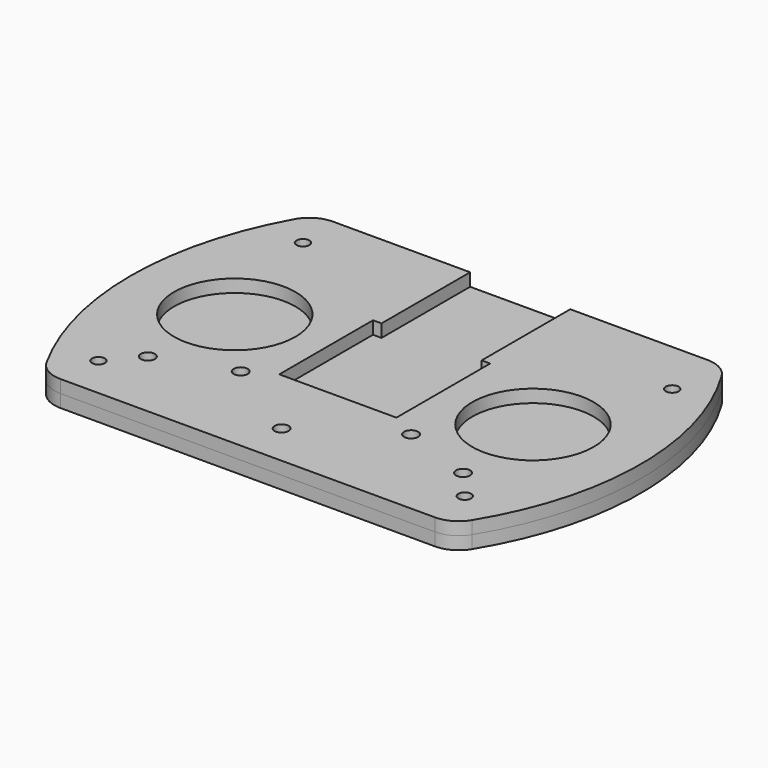
from build123d import *

# Parameters (mm, degrees)
F0_R     = 1.5
F1_DEPTH = 3
F2_DEPTH = 3
F3_R     = 14.25
F3_R_2   = 1.65
F4_DEPTH = 25
F6_DEPTH = 3
F7_DEPTH = 3
F8_W     = 23.5
F8_H     = 37.6963340342
F9_DEPTH = 25


with BuildPart() as f1:
    # F0 (on Top) → F1 (new body)
    with BuildSketch(Plane.XY):
        with BuildLine():
            Line((45.1, 35), (-45.1, 35))
            ThreePointArc((-45.1, 35), (-54.4782217351, 0), (-45.1, -35))
            Line((-45.1, -35), (45.1, -35))
            ThreePointArc((45.1, -35), (55.2720579016, 0), (45.1, 35))
        make_face()
        with Locations((-43, -30)):
            Circle(F0_R, mode=Mode.SUBTRACT)
        with Locations((43, -30)):
            Circle(F0_R, mode=Mode.SUBTRACT)
        with Locations((-43, 30)):
            Circle(F0_R, mode=Mode.SUBTRACT)
        with Locations((46.13, 26.95)):
            Circle(F0_R, mode=Mode.SUBTRACT)
    extrude(amount=-F1_DEPTH)

    # F5 (on Top) → F6 (join)
    with BuildSketch(Plane.XY):
        with BuildLine():
            ThreePointArc((-50.0545445124, 36.3970588235), (-59.4782217351, 0), (-50.0545445124, -36.3970588235))
            ThreePointArc((-50.0545445124, -36.3970588235), (-47.4851853132, -39.0323880746), (-43.9340877199, -40))
            Line((-43.9340877199, -40), (43.9895550669, -40))
            ThreePointArc((43.9895550669, -40), (47.4140971022, -39.1051217718), (49.9630539635, -36.6492890995))
            ThreePointArc((49.9630539635, -36.6492890995), (60.2720579016, 0), (49.9630539635, 36.6492890995))
            ThreePointArc((49.9630539635, 36.6492890995), (47.4140971022, 39.1051217718), (43.9895550669, 40))
            Line((43.9895550669, 40), (-43.9340877199, 40))
            ThreePointArc((-43.9340877199, 40), (-47.4851853132, 39.0323880746), (-50.0545445124, 36.3970588235))
        make_face()
        with BuildLine():
            Line((44.5476018751, -34), (-44.5198739442, -34))
            ThreePointArc((-44.5198739442, -34), (-53.4782217351, 0), (-44.5198739442, 34))
            Line((-44.5198739442, 34), (44.5476018751, 34))
            ThreePointArc((44.5476018751, 34), (54.2720579016, 0), (44.5476018751, -34))
        make_face(mode=Mode.SUBTRACT)
    extrude(amount=-F6_DEPTH)


with BuildPart() as f2:
    # F0 (on Top) → F2 (new body)
    with BuildSketch(Plane.XY):
        with BuildLine():
            Line((45.1, 35), (-45.1, 35))
            ThreePointArc((-45.1, 35), (-54.4782217351, 0), (-45.1, -35))
            Line((-45.1, -35), (45.1, -35))
            ThreePointArc((45.1, -35), (55.2720579016, 0), (45.1, 35))
        make_face()
        with Locations((-43, -30)):
            Circle(F0_R, mode=Mode.SUBTRACT)
        with Locations((43, -30)):
            Circle(F0_R, mode=Mode.SUBTRACT)
        with Locations((-43, 30)):
            Circle(F0_R, mode=Mode.SUBTRACT)
        with Locations((46.13, 26.95)):
            Circle(F0_R, mode=Mode.SUBTRACT)
    extrude(amount=F2_DEPTH)

    # F3 (on Top) → F4 (cut)
    with BuildSketch(Plane.XY):
        Polygon((-11.75, 14), (-13.75, 14), (-13.75, -13.5), (13.75, -13.5), (13.75, 14), (11.75, 14), (11.75, 43.5743890703), (-11.75, 43.5743890703), align=None)
        with Locations((-35, 0)):
            Circle(F3_R)
        with Locations((35, 0)):
            Circle(F3_R)
        with Locations((-37, -23)):
            Circle(F3_R_2)
        with Locations((-20, -17)):
            Circle(F3_R_2)
        with Locations((0, -30)):
            Circle(F3_R_2)
        with Locations((37, -23)):
            Circle(F3_R_2)
        with Locations((20, -17)):
            Circle(F3_R_2)
    extrude(amount=F4_DEPTH, mode=Mode.SUBTRACT)

    # F5 (on Top) → F7 (join)
    with BuildSketch(Plane.XY):
        with BuildLine():
            ThreePointArc((-50.0545445124, 36.3970588235), (-59.4782217351, 0), (-50.0545445124, -36.3970588235))
            ThreePointArc((-50.0545445124, -36.3970588235), (-47.4851853132, -39.0323880746), (-43.9340877199, -40))
            Line((-43.9340877199, -40), (43.9895550669, -40))
            ThreePointArc((43.9895550669, -40), (47.4140971022, -39.1051217718), (49.9630539635, -36.6492890995))
            ThreePointArc((49.9630539635, -36.6492890995), (60.2720579016, 0), (49.9630539635, 36.6492890995))
            ThreePointArc((49.9630539635, 36.6492890995), (47.4140971022, 39.1051217718), (43.9895550669, 40))
            Line((43.9895550669, 40), (-43.9340877199, 40))
            ThreePointArc((-43.9340877199, 40), (-47.4851853132, 39.0323880746), (-50.0545445124, 36.3970588235))
        make_face()
        with BuildLine():
            Line((44.5476018751, -34), (-44.5198739442, -34))
            ThreePointArc((-44.5198739442, -34), (-53.4782217351, 0), (-44.5198739442, 34))
            Line((-44.5198739442, 34), (44.5476018751, 34))
            ThreePointArc((44.5476018751, 34), (54.2720579016, 0), (44.5476018751, -34))
        make_face(mode=Mode.SUBTRACT)
    extrude(amount=F7_DEPTH)

    # F8 (on face) → F9 (cut)
    with BuildSketch(Plane.XY.offset(3)):
        with Locations((0, 32.8481670171)):
            Rectangle(F8_W, F8_H)
    extrude(amount=-F9_DEPTH, mode=Mode.SUBTRACT)


solid = Compound([f1.part, f2.part])
